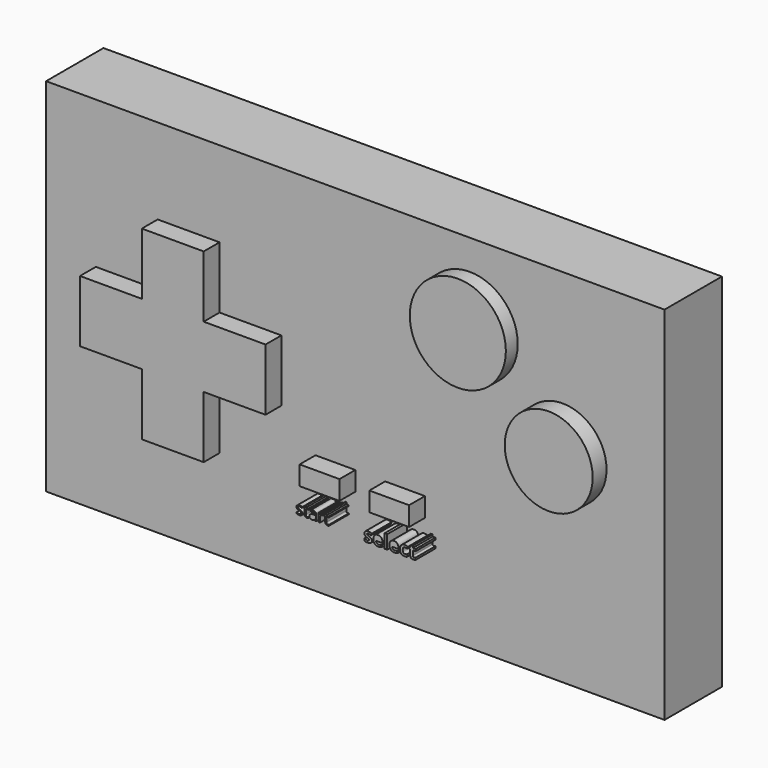
from build123d import *

# Parameters (mm, degrees)
F0_W           = 63.5
F0_H           = 37.0902135537
F0_R           = 4.5160291378
F0_R_2         = 4.9339168697
F1_DEPTH       = 7.366
F3_DEPTH       = 8.89
F4_DEPTH       = 9.144
F5_W           = 4.0797665715
F5_H           = 1.9707353786
F5_W_2         = 4.0894
F6_DEPTH       = 9.398
F7_TEXT_SIZE   = 1.8403360931
F7_TEXT_SIZE_2 = 1.6073334134
F9_DEPTH       = 2.54


# Not quite as in the source:
# - Text() gives the source's letters only with a copy of the font that has no kerning and outlines rounded to 1/6400 em; it was checked with that copy


with BuildPart() as f1:
    # F0 (on Front) → F1 (new body)
    with BuildSketch(Plane.XZ):
        with Locations((31.75, 18.5451067768)):
            Rectangle(F0_W, F0_H)
        with Locations((53.0298836529, 20.7002628595)):
            Circle(F0_R, mode=Mode.SUBTRACT)
        with Locations((43.4938110411, 29.0734004229)):
            Circle(F0_R_2, mode=Mode.SUBTRACT)
    extrude(amount=F1_DEPTH)

    # F0 (on Front) → F3 (join)
    with BuildSketch(Plane.XZ):
        with Locations((43.4938110411, 29.0734004229)):
            Circle(F0_R_2)
    extrude(amount=F3_DEPTH)

    # F0 (on Front) → F4 (join)
    with BuildSketch(Plane.XZ):
        with Locations((53.0298836529, 20.7002628595)):
            Circle(F0_R)
    extrude(amount=F4_DEPTH)

    # F5 (on Front) → F6 (join)
    with BuildSketch(Plane.XZ):
        with Locations((36.8574298918, 11.2516512163)):
            Rectangle(F5_W, F5_H)
        Polygon((17.8083269089, 28.3177030876), (11.4583269089, 28.3177030876), (11.4583269089, 21.9677030876), (5.1083269089, 21.9677030876), (5.1083269089, 15.6177030876), (11.4583269089, 15.6177030876), (11.4583269089, 9.2677030876), (17.8083269089, 9.2677030876), (17.8083269089, 15.6177030876), (24.1583269089, 15.6177030876), (24.1583269089, 21.9677030876), (17.8083269089, 21.9677030876), align=None)
        with Locations((29.7053678963, 11.2862256356)):
            Rectangle(F5_W_2, F5_H)
    extrude(amount=F6_DEPTH)

    # F7 (on face) → F9 (join)
    with BuildSketch(Plane.XZ.offset(7.366)):
        with Locations((34.6390455961, 7.8213699162)):
            Text('select', F7_TEXT_SIZE, font='Open Sans', font_style=FontStyle.BOLD, text_align=(TextAlign.LEFT, TextAlign.BOTTOM))
        with Locations((27.6606678963, 8.0280741677)):
            Text('start', F7_TEXT_SIZE_2, font='Open Sans', text_align=(TextAlign.LEFT, TextAlign.BOTTOM))
        with BuildLine():
            add(Edge.make_bspline(
                [(29.247909642, 8.1567864137), (29.2906044358, 8.1199935472), (29.3674550647, 8.1199935472)],
                knots=[0, 0, 0, 1, 1, 1], degree=2))
            add(Edge.make_bspline(
                [(29.3674550647, 8.1199935472), (29.4892607999, 8.1199935472), (29.5587026263, 8.1866727693)],
                knots=[0, 0, 0, 1, 1, 1], degree=2))
            add(Edge.make_bspline(
                [(29.5587026263, 8.1866727693), (29.6281444526, 8.2533519914), (29.6281444526, 8.3733997057)],
                knots=[0, 0, 0, 1, 1, 1], degree=2))
            Line((29.6281444526, 8.3733997057), (29.6281444526, 8.4510037721))
            Line((29.6281444526, 8.4510037721), (29.4977997587, 8.4457297093))
            add(Edge.make_bspline(
                [(29.4977997587, 8.4457297093), (29.3423404801, 8.4402045007), (29.2737776642, 8.397384134)],
                knots=[0, 0, 0, 1, 1, 1], degree=2))
            add(Edge.make_bspline(
                [(29.2737776642, 8.397384134), (29.2052148482, 8.3545637673), (29.2052148482, 8.2644024086)],
                knots=[0, 0, 0, 1, 1, 1], degree=2))
            add(Edge.make_bspline(
                [(29.2052148482, 8.2644024086), (29.2052148482, 8.1935792801), (29.247909642, 8.1567864137)],
                knots=[0, 0, 0, 1, 1, 1], degree=2))
        make_face()
        with BuildLine():
            add(Edge.make_bspline(
                [(37.9007537686, 8.5945986278), (37.849569421, 8.6498087106), (37.7624410091, 8.6498087106)],
                knots=[0, 0, 0, 1, 1, 1], degree=2))
            add(Edge.make_bspline(
                [(37.7624410091, 8.6498087106), (37.6753125972, 8.6498087106), (37.6258535647, 8.5945986278)],
                knots=[0, 0, 0, 1, 1, 1], degree=2))
            add(Edge.make_bspline(
                [(37.6258535647, 8.5945986278), (37.5763945322, 8.539388545), (37.5692057193, 8.4378825074)],
                knots=[0, 0, 0, 1, 1, 1], degree=2))
            Line((37.5692057193, 8.4378825074), (37.9539509837, 8.4378825074))
            add(Edge.make_bspline(
                [(37.9539509837, 8.4378825074), (37.9519381161, 8.539388545), (37.9007537686, 8.5945986278)],
                knots=[0, 0, 0, 1, 1, 1], degree=2))
        make_face()
        with BuildLine():
            add(Edge.make_bspline(
                [(36.2519276502, 8.5945986278), (36.2007433026, 8.6498087106), (36.1136148907, 8.6498087106)],
                knots=[0, 0, 0, 1, 1, 1], degree=2))
            add(Edge.make_bspline(
                [(36.1136148907, 8.6498087106), (36.0264864788, 8.6498087106), (35.9770274463, 8.5945986278)],
                knots=[0, 0, 0, 1, 1, 1], degree=2))
            add(Edge.make_bspline(
                [(35.9770274463, 8.5945986278), (35.9275684138, 8.539388545), (35.9203796009, 8.4378825074)],
                knots=[0, 0, 0, 1, 1, 1], degree=2))
            Line((35.9203796009, 8.4378825074), (36.3051248654, 8.4378825074))
            add(Edge.make_bspline(
                [(36.3051248654, 8.4378825074), (36.3031119978, 8.539388545), (36.2519276502, 8.5945986278)],
                knots=[0, 0, 0, 1, 1, 1], degree=2))
        make_face()
    extrude(amount=F9_DEPTH)


solid = f1.part
